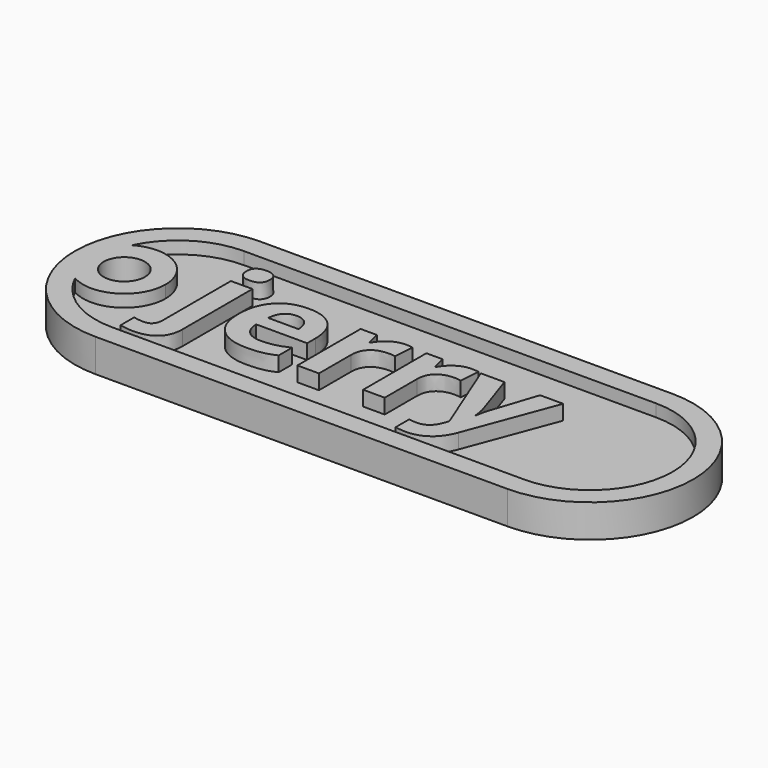
from build123d import *

# Parameters (mm, degrees)
F1_DEPTH     = 4
F3_DEPTH     = 1.5
F6_DEPTH     = 1.5
F7_R         = 2.5
F8_DEPTH     = 25
F9_TEXT_SIZE = 17.5638699956
F10_DEPTH    = 1.8


# Not quite as in the source:
# - Text() gives the source's letters only with a copy of the font that has no kerning and outlines rounded to 1/6400 em; it was checked with that copy


with BuildPart() as f1:
    # F0 (on Top) → F1 (new body)
    with BuildSketch(Plane.XY):
        with BuildLine():
            ThreePointArc((12.5, 25), (0, 12.5), (12.5, 0))
            Line((12.5, 0), (62.5, 0))
            ThreePointArc((62.5, 0), (75, 12.5), (62.5, 25))
            Line((62.5, 25), (12.5, 25))
        make_face()
    extrude(amount=F1_DEPTH)

    # F2 (on face) → F3 (cut)
    with BuildSketch(Plane.XY.offset(4)):
        with BuildLine():
            Line((62.5, 22.5), (12.5, 22.5))
            ThreePointArc((12.5, 22.5), (2.5, 12.5), (12.5, 2.5))
            Line((12.5, 2.5), (62.5, 2.5))
            ThreePointArc((62.5, 2.5), (72.5, 12.5), (62.5, 22.5))
        make_face()
    extrude(amount=-F3_DEPTH, mode=Mode.SUBTRACT)

    # F4 (on face) → F6 (join)
    with BuildSketch(Plane.XY.offset(2.5)):
        with BuildLine():
            ThreePointArc((3.4807692308, 8.1810329555), (8.4903660528, 8.1643250902), (11, 12.5))
            ThreePointArc((11, 12.5), (8.4903660528, 16.8356749098), (3.4807692308, 16.8189670445))
            ThreePointArc((3.4807692308, 16.8189670445), (2.5, 12.5), (3.4807692308, 8.1810329555))
        make_face()
    extrude(amount=F6_DEPTH)

    # F7 (on face) → F8 (cut)
    with BuildSketch(Plane.XY.offset(4)):
        with Locations((6, 12.5)):
            Circle(F7_R)
    extrude(amount=-F8_DEPTH, mode=Mode.SUBTRACT)

    # F9 (on face) → F10 (join)
    with BuildSketch(Plane.XY.offset(2.5)):
        with Locations((14.3677759916, 6.8978103809)):
            Text('jerry', F9_TEXT_SIZE, font='Open Sans', font_style=FontStyle.BOLD, text_align=(TextAlign.LEFT, TextAlign.BOTTOM))
    extrude(amount=F10_DEPTH)


solid = f1.part
